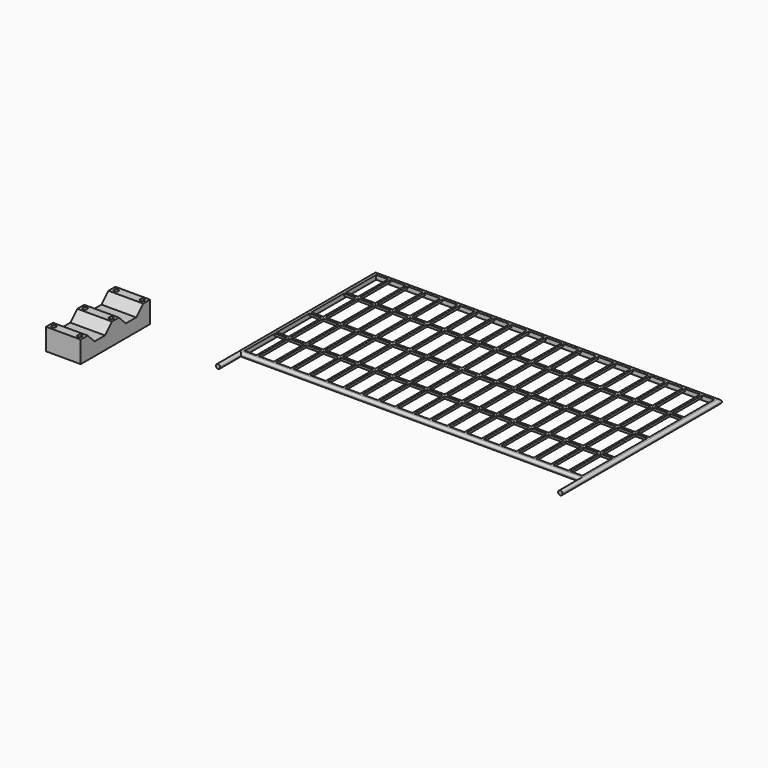
from build123d import *

# Parameters (mm, degrees)
F0_W      = 78
F0_H      = 38
F0_W_2    = 1
F0_H_2    = 6
F1_DEPTH  = 1
F2_W      = 0.5
F2_H      = 38
F3_DEPTH  = 0.5
F4_W      = 3.5
F4_H      = 0.5997701301
F4_W_2    = 2.75
F4_H_2    = 0.6
F4_W_3    = 2.730001321
F5_DEPTH  = 0.5
F6_R      = 0.49999
F7_W      = 8
F7_H      = 20
F7_R      = 0.5
F8_DEPTH  = 5
F10_DEPTH = 25


# Not quite as in the source:
# - a fillet or chamfer is up to 0.001 mm smaller than in the source, because OpenCascade refuses the exact size


with BuildPart() as f1:
    # F0 (on Top) → F1 (new body)
    with BuildSketch(Plane.XY):
        Polygon((0, 40), (0, 0), (1, 0), (79, 0), (80, 0), (80, 40), align=None)
        with Locations((40, 20)):
            Rectangle(F0_W, F0_H, mode=Mode.SUBTRACT)
        with Locations((0.5, -3)):
            Rectangle(F0_W_2, F0_H_2)
        with Locations((79.5, -3)):
            Rectangle(F0_W_2, F0_H_2)
    extrude(amount=F1_DEPTH)

    # F2 (on face) → F3 (join)
    with BuildSketch(Plane.XY.offset(1)):
        with Locations((40, 20)):
            Rectangle(F2_W, F2_H)
        with Locations((44, 20)):
            Rectangle(F2_W, F2_H)
        with Locations((48, 20)):
            Rectangle(F2_W, F2_H)
        with Locations((52, 20)):
            Rectangle(F2_W, F2_H)
        with Locations((56, 20)):
            Rectangle(F2_W, F2_H)
        with Locations((60, 20)):
            Rectangle(F2_W, F2_H)
        with Locations((64, 20)):
            Rectangle(F2_W, F2_H)
        with Locations((68, 20)):
            Rectangle(F2_W, F2_H)
        with Locations((72, 20)):
            Rectangle(F2_W, F2_H)
        with Locations((76, 20)):
            Rectangle(F2_W, F2_H)
        with Locations((36, 20)):
            Rectangle(F2_W, F2_H)
        with Locations((32, 20)):
            Rectangle(F2_W, F2_H)
        with Locations((28, 20)):
            Rectangle(F2_W, F2_H)
        with Locations((24, 20)):
            Rectangle(F2_W, F2_H)
        with Locations((20, 20)):
            Rectangle(F2_W, F2_H)
        with Locations((16, 20)):
            Rectangle(F2_W, F2_H)
        with Locations((12, 20)):
            Rectangle(F2_W, F2_H)
        with Locations((8, 20)):
            Rectangle(F2_W, F2_H)
        with Locations((4, 20)):
            Rectangle(F2_W, F2_H)
    extrude(amount=-F3_DEPTH)

    # F4 (on face) → F5 (join)
    with BuildSketch(Plane.XY.offset(1)):
        with Locations((10, 29.9998850651)):
            Rectangle(F4_W, F4_H)
        with Locations((6, 29.9998850651)):
            Rectangle(F4_W, F4_H)
        with Locations((2.375, 29.9998850651)):
            Rectangle(F4_W_2, F4_H)
        with Locations((14, 29.9998850651)):
            Rectangle(F4_W, F4_H)
        with Locations((18, 29.9998850651)):
            Rectangle(F4_W, F4_H)
        with Locations((22, 29.9998850651)):
            Rectangle(F4_W, F4_H)
        with Locations((26, 29.9998850651)):
            Rectangle(F4_W, F4_H)
        with Locations((30, 29.9998850651)):
            Rectangle(F4_W, F4_H)
        with Locations((34, 29.9998850651)):
            Rectangle(F4_W, F4_H)
        with Locations((38, 29.9998850651)):
            Rectangle(F4_W, F4_H)
        with Locations((42, 29.9998850651)):
            Rectangle(F4_W, F4_H)
        with Locations((46, 29.9998850651)):
            Rectangle(F4_W, F4_H)
        with Locations((50, 29.9998850651)):
            Rectangle(F4_W, F4_H)
        with Locations((54, 29.9998850651)):
            Rectangle(F4_W, F4_H)
        with Locations((58, 29.9998850651)):
            Rectangle(F4_W, F4_H)
        with Locations((62, 29.9998850651)):
            Rectangle(F4_W, F4_H)
        with Locations((66, 29.9998850651)):
            Rectangle(F4_W, F4_H)
        with Locations((70, 29.9998850651)):
            Rectangle(F4_W, F4_H)
        Polygon((76.25, 29.7), (79, 29.7), (79, 30.3), (76.25, 30.3), (76.25, 30.2998850651), (76.25, 30.2997701301), align=None)
        with Locations((74, 29.9998850651)):
            Rectangle(F4_W, F4_H)
        Polygon((79, 20.3), (76.25, 20.3), (76.25, 20.2998850651), (76.25, 20.2997701301), (76.25, 19.7), (79, 19.7), align=None)
        with Locations((74, 19.9998850651)):
            Rectangle(F4_W, F4_H)
        with Locations((70, 19.9998850651)):
            Rectangle(F4_W, F4_H)
        with Locations((66, 19.9998850651)):
            Rectangle(F4_W, F4_H)
        with Locations((62, 19.9998850651)):
            Rectangle(F4_W, F4_H)
        with Locations((58, 19.9998850651)):
            Rectangle(F4_W, F4_H)
        with Locations((54, 19.9998850651)):
            Rectangle(F4_W, F4_H)
        with Locations((50, 19.9998850651)):
            Rectangle(F4_W, F4_H)
        with Locations((46, 19.9998850651)):
            Rectangle(F4_W, F4_H)
        with Locations((42, 19.9998850651)):
            Rectangle(F4_W, F4_H)
        with Locations((38, 19.9998850651)):
            Rectangle(F4_W, F4_H)
        with Locations((34, 19.9998850651)):
            Rectangle(F4_W, F4_H)
        with Locations((30, 19.9998850651)):
            Rectangle(F4_W, F4_H)
        with Locations((26, 19.9998850651)):
            Rectangle(F4_W, F4_H)
        with Locations((22, 19.9998850651)):
            Rectangle(F4_W, F4_H)
        with Locations((18, 19.9998850651)):
            Rectangle(F4_W, F4_H)
        with Locations((14, 19.9998850651)):
            Rectangle(F4_W, F4_H)
        with Locations((10, 19.9998850651)):
            Rectangle(F4_W, F4_H)
        with Locations((6, 19.9998850651)):
            Rectangle(F4_W, F4_H)
        with Locations((2.375, 19.9998850651)):
            Rectangle(F4_W_2, F4_H)
        with Locations((6, 10.0002298699)):
            Rectangle(F4_W, F4_H_2)
        with Locations((2.375, 10.0002298699)):
            Rectangle(F4_W_2, F4_H_2)
        with Locations((10, 10.0002298699)):
            Rectangle(F4_W, F4_H_2)
        with Locations((14, 10.0002298699)):
            Rectangle(F4_W, F4_H_2)
        with Locations((18, 10.0002298699)):
            Rectangle(F4_W, F4_H_2)
        with Locations((22, 10.0002298699)):
            Rectangle(F4_W, F4_H_2)
        with Locations((26, 10.0002298699)):
            Rectangle(F4_W, F4_H_2)
        with Locations((30, 10.0002298699)):
            Rectangle(F4_W, F4_H_2)
        with Locations((34, 10.0002298699)):
            Rectangle(F4_W, F4_H_2)
        with Locations((38, 10.0002298699)):
            Rectangle(F4_W, F4_H_2)
        with Locations((42, 10.0002298699)):
            Rectangle(F4_W, F4_H_2)
        with Locations((46, 10.0002298699)):
            Rectangle(F4_W, F4_H_2)
        with Locations((50, 10.0002298699)):
            Rectangle(F4_W, F4_H_2)
        with Locations((54, 10.0002298699)):
            Rectangle(F4_W, F4_H_2)
        with Locations((58, 10.0002298699)):
            Rectangle(F4_W, F4_H_2)
        with Locations((62, 10.0002298699)):
            Rectangle(F4_W, F4_H_2)
        with Locations((66, 10.0002298699)):
            Rectangle(F4_W, F4_H_2)
        with Locations((70, 10.0002298699)):
            Rectangle(F4_W, F4_H_2)
        with Locations((74, 10.0002298699)):
            Rectangle(F4_W, F4_H_2)
        with Locations((77.6150006605, 10.0002298699)):
            Rectangle(F4_W_3, F4_H_2)
    extrude(amount=-F5_DEPTH)

    # F6 (radius 0.5 in the source; OpenCascade refuses exactly that, so slightly less here)
    f6_edges = [f1.edges().sort_by_distance(p)[0] for p in [
        (80, 17, 1),
        (80, 17, 0),
        (79, -3, 1),
        (79, -3, 0),
        (40, 0, 1),
        (40, 0, 0),
        (0, 17, 1),
        (0, 17, 0),
        (1, -3, 0),
        (1, -3, 1),
        (40, 40, 1),
        (40, 40, 0),
    ]]
    fillet(f6_edges, radius=F6_R)


with BuildPart() as f8:
    # F7 (on Top) → F8 (new body)
    with BuildSketch(Plane.XY):
        with Locations((-24, -10)):
            Rectangle(F7_W, F7_H)
        with Locations((-27, -19)):
            Circle(F7_R, mode=Mode.SUBTRACT)
        with Locations((-21, -19)):
            Circle(F7_R, mode=Mode.SUBTRACT)
        with Locations((-27, -10)):
            Circle(F7_R, mode=Mode.SUBTRACT)
        with Locations((-27, -1)):
            Circle(F7_R, mode=Mode.SUBTRACT)
        with Locations((-21, -10)):
            Circle(F7_R, mode=Mode.SUBTRACT)
        with Locations((-21, -1)):
            Circle(F7_R, mode=Mode.SUBTRACT)
    extrude(amount=F8_DEPTH)

    # F9 (on face) → F10 (cut)
    with BuildSketch(Plane(origin=(-28, 0, 0), x_dir=(0, -1, 0), z_dir=(-1, 0, 0))):
        Polygon((9, 5), (2, 5), (4, 3), (7, 3), align=None)
        Polygon((18, 5), (11, 5), (13, 3), (16, 3), align=None)
    extrude(amount=-F10_DEPTH, mode=Mode.SUBTRACT)


solid = Compound([f1.part, f8.part])
